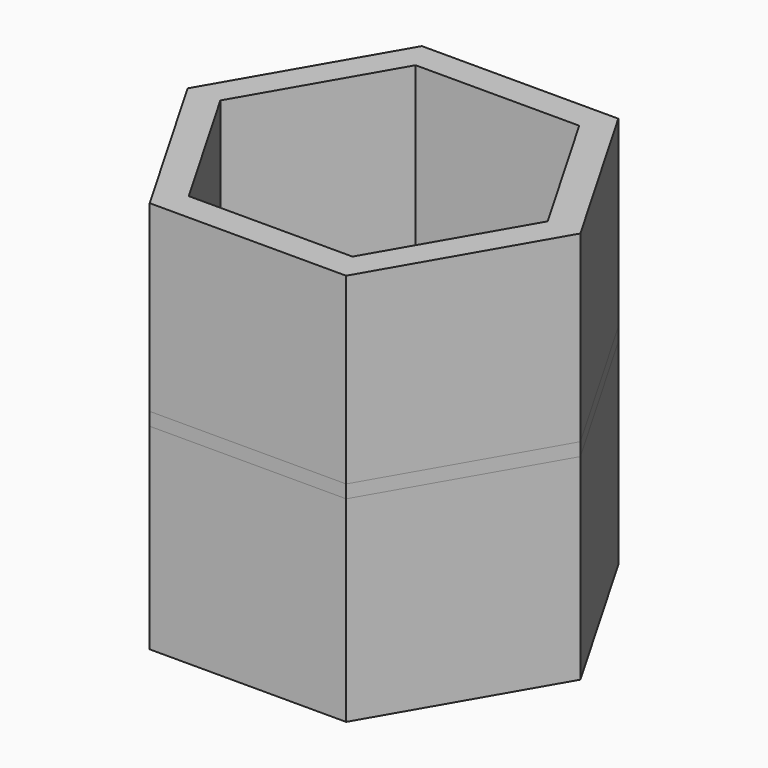
from build123d import *

# Parameters (mm, degrees)
F1_DEPTH  = 30
F4_DEPTH  = 2
F6_DEPTH  = 4
F7_DEPTH  = 2
F13_DEPTH = 24.5
F15_DEPTH = 24.7
F16_DEPTH = 2
F17_DEPTH = 2
F20_DEPTH = 2
F22_W     = 20.7
F22_H     = 21.2839984947
F23_DEPTH = 1.9791820473


with BuildPart() as f1:
    # F0 (on Top) → F1 (new body, symmetric)
    with BuildSketch(Plane.XY):
        Polygon((15, -25.9807621135), (30, 0), (15, 25.9807621135), (-15, 25.9807621135), (-30, 0), (-15, -25.9807621135), align=None)
        Polygon((-12.5, -21.6506350946), (-25, 0), (-12.5, 21.6506350946), (12.5, 21.6506350946), (25, 0), (12.5, -21.6506350946), align=None, mode=Mode.SUBTRACT)
    extrude(amount=F1_DEPTH, both=True)

    # F3 (on 3pt) → F4 (join)
    with BuildSketch(Plane(origin=(0, 0, -30), x_dir=(1, 0, 0), z_dir=(0, 0, -1))):
        Polygon((-25, 0), (-12.5, -21.6506350946), (12.5, -21.6506350946), (25, 0), (12.5, 21.6506350946), (-12.5, 21.6506350946), align=None)
    extrude(amount=-F4_DEPTH)


with BuildPart() as f6:
    # F5 (on Top) → F6 (new body)
    with BuildSketch(Plane.XY):
        Polygon((-12.45, 21.5640325542), (-24.9, 0), (-12.45, -21.5640325542), (12.45, -21.5640325542), (24.9, 0), (12.45, 21.5640325542), align=None)
    extrude(amount=-F6_DEPTH)

    # F5 (on Top) → F7 (join)
    with BuildSketch(Plane.XY):
        Polygon((15, -25.9807621135), (30, 0), (15, 25.9807621135), (-15, 25.9807621135), (-30, 0), (-15, -25.9807621135), align=None)
        Polygon((-12.45, -21.5640325542), (-24.9, 0), (-12.45, 21.5640325542), (12.45, 21.5640325542), (24.9, 0), (12.45, -21.5640325542), align=None, mode=Mode.SUBTRACT)
        Polygon((-12.45, 21.5640325542), (-24.9, 0), (-12.45, -21.5640325542), (12.45, -21.5640325542), (24.9, 0), (12.45, 21.5640325542), align=None)
    extrude(amount=F7_DEPTH)


with BuildPart() as f13:
    # F12 (on 3pt) → F13 (new body)
    with BuildSketch(Plane(origin=(-12.25, 0, 0), x_dir=(0, -1, 0), z_dir=(-1, 0, 0))):
        Polygon((6.5, 0), (-6.5, 0), (-1.75, -25), (1.75, -25), align=None)
    extrude(amount=-F13_DEPTH)


with BuildPart() as f15:
    # F14 (on 3pt) → F15 (new body)
    with BuildSketch(Plane(origin=(-12.25, 0, 0), x_dir=(0, -1, 0), z_dir=(-1, 0, 0))):
        Polygon((-6.321952302, -22.0473393536), (-11.073605489, 2.9613616306), (-13.073605489, 2.9613616306), (-7.9407595883, -24.0536167943), (0, -24.0386383694), (3.926394511, 2.9613616306), (1.926394511, 2.9613616306), (-1.7091559621, -22.0386383694), align=None)
    extrude(amount=-F15_DEPTH)

    # F16 (add): a face of the model
    f16_faces = [f15.faces().sort_by_distance(p)[0] for p in [
        (-12.25, -0.4244847403, -9.5845721632),
    ]]
    extrude(f16_faces, amount=F16_DEPTH)

    # F14 (on 3pt) → F17 (join)
    with BuildSketch(Plane(origin=(-12.25, 0, 0), x_dir=(0, -1, 0), z_dir=(-1, 0, 0))):
        Polygon((1.926394511, 2.9613616306), (-11.073605489, 2.9613616306), (-6.321952302, -22.0473393536), (-1.7091559621, -22.0386383694), align=None)
        Polygon((-6.321952302, -22.0473393536), (-11.073605489, 2.9613616306), (-13.073605489, 2.9613616306), (-7.9407595883, -24.0536167943), (0, -24.0386383694), (3.926394511, 2.9613616306), (1.926394511, 2.9613616306), (-1.7091559621, -22.0386383694), align=None)
    extrude(amount=F17_DEPTH)

    # F19 (on 3pt) → F20 (join)
    with BuildSketch(Plane(origin=(12.45, 0, 0), x_dir=(0, -1, 0), z_dir=(-1, 0, 0))):
        Polygon((3.926394511, 2.9613616306), (-13.073605489, 2.9613616306), (-7.9407595883, -24.0536167943), (0, -24.0386383694), align=None)
    extrude(amount=-F20_DEPTH)

    # F22 (on 3pt) → F23 (cut, through all)
    with BuildSketch(Plane(origin=(0, -3.4233517746, -0.4978307266), x_dir=(1, 0, 0), z_dir=(0, -0.9895910237, -0.1439083246))):
        with Locations((0.1, -9.1464215042)):
            Rectangle(F22_W, F22_H)
    extrude(amount=-F23_DEPTH, mode=Mode.SUBTRACT)


solid = Compound([f1.part, f6.part, f13.part, f15.part])
